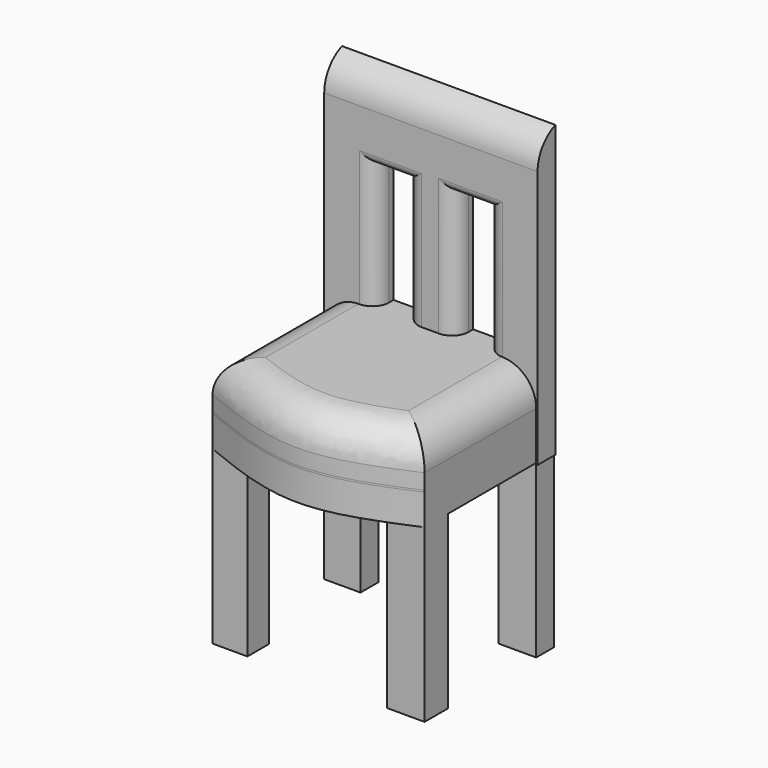
from build123d import *

# Parameters (mm, degrees)
F0_W        = 31.6318599507
F0_H        = 42.7960464731
F0_W_2      = 4.3416279368
F0_H_2      = 18.813719973
F0_W_3      = 4.5483717695
F0_H_3      = 19.0204642713
F1_DEPTH    = 3.302
F3_DEPTH    = 0.254
F4_DEPTH    = 12.192
F5_DEPTH    = 7.62
F6_DEPTH    = 7.366
F7_R        = 5.08
F8_T1_DEPTH = 55.4253023246
F9_W        = 5.16293291
F9_H        = 4.0333122015
F9_W_2      = 5.5523253977
F9_H_2      = 4.3130330741
F9_H_3      = 3.302
F9_W_3      = 5.3753489628
F10_DEPTH   = 25.4
F11_R       = 2.4528409794
F12_R       = 1.2264204897


# Not quite as in the source:
# - a fillet or chamfer that OpenCascade refuses, or shapes differently, is made with other operations: its cross-section is extruded or revolved along the edge and cut away or added


with BuildPart() as f1:
    # F0 (on Front) → F1 (new body)
    with BuildSketch(Plane.XZ):
        with Locations((-0.3101159818, 8.9933718555)):
            Rectangle(F0_W, F0_H)
        with Locations((-6.3056976069, 9.4068599865)):
            Rectangle(F0_W_2, F0_H_2, mode=Mode.SUBTRACT)
        with Locations((5.5820937268, 9.5102321357)):
            Rectangle(F0_W_3, F0_H_3, mode=Mode.SUBTRACT)
    extrude(amount=F1_DEPTH)

    # F3 (add): a face of the model
    f3_faces = [f1.faces().sort_by_distance(p)[0] for p in [
        (-0.3101159818, -1.651, 30.391395092),
    ]]
    extrude(f3_faces, amount=F3_DEPTH)

    # F2 (on Top) → F4 (join)
    with BuildSketch(Plane.XY):
        with BuildLine():
            Line((-16.1260459572, -3.0640123878), (-16.1260459572, -5.3753489628))
            Line((-16.1260459572, -5.3753489628), (-16.1260459572, -23.9823255688))
            add(Edge.make_bspline(
                [(-16.1260459572, -23.9823255688), (-10.712885637, -26.1710511495), (-0.0173269949, -30.4956307693), (10.2353861269, -26.1356592233), (15.2990687639, -23.9823255688)],
                knots=[0, 0, 0, 0, 0.5061129111, 1, 1, 1, 1], degree=3))
            Line((15.2990687639, -23.9823255688), (15.2990687639, -5.1686046645))
            Line((15.2990687639, -5.1686046645), (15.2990687639, -3.0640123878))
            Line((15.2990687639, -3.0640123878), (-16.1260459572, -3.0640123878))
        make_face()
    extrude(amount=-F4_DEPTH)

    # F5 (add): a face of the model
    f5_faces = [f1.faces().sort_by_distance(p)[0] for p in [
        (-0.3946759913, -14.5235842944, 0),
    ]]
    extrude(f5_faces, amount=-F5_DEPTH)

    # F6 (add): a face of the model
    f6_faces = [f1.faces().sort_by_distance(p)[0] for p in [
        (-0.3946759913, -14.5235842944, 0),
    ]]
    extrude(f6_faces, amount=-F6_DEPTH)

    # F7
    f7_edges = [f1.edges().sort_by_distance(p)[0] for p in [
        (-0.398964, -28.322485, 0),
        (15.299069, -13.642163, 0),
        (-16.126046, -13.642163, 0),
    ]]
    fillet(f7_edges, radius=F7_R)

    # F8: fillet of radius 5.08 on 1 edges, made by hand

    # F8_s2 → F8_t1 (cut)
    with BuildSketch(Plane.YZ.offset(-28.0227671442)):
        with BuildLine():
            ThreePointArc((-3.302, 25.8867066172), (-2.3956458882, 28.782752197), (0, 30.645395092))
            Line((0, 30.645395092), (-3.302, 30.645395092))
            Line((-3.302, 30.645395092), (-3.302, 25.8867066172))
        make_face()
    extrude(amount=F8_T1_DEPTH, mode=Mode.SUBTRACT)

    # F9 (on face) → F10 (join)
    with BuildSketch(Plane(origin=(0, 0, -12.192), x_dir=(1, 0, 0), z_dir=(0, 0, -1))):
        with Locations((-13.5445795022, 21.965669468)):
            Rectangle(F9_W, F9_H)
        with Locations((12.522906065, 21.8258090317)):
            Rectangle(F9_W_2, F9_H_2)
        with Locations((12.522906065, 1.651)):
            Rectangle(F9_W_2, F9_H_3)
        with Locations((-13.4383714758, 1.651)):
            Rectangle(F9_W_3, F9_H_3)
    extrude(amount=F10_DEPTH)

    # F11
    f11_edges = [f1.edges().sort_by_distance(p)[0] for p in [
        (-8.476512, -3.302, 9.40686),
        (7.85628, -3.302, 9.510232),
        (3.307908, -3.302, 9.510232),
        (-4.134884, -3.302, 9.40686),
    ]]
    fillet(f11_edges, radius=F11_R)

    # F12
    f12_edges = [f1.edges().sort_by_distance(p)[0] for p in [
        (5.582094, -3.302, 19.020464),
        (-6.305698, -3.302, 18.81372),
    ]]
    fillet(f12_edges, radius=F12_R)


solid = f1.part
